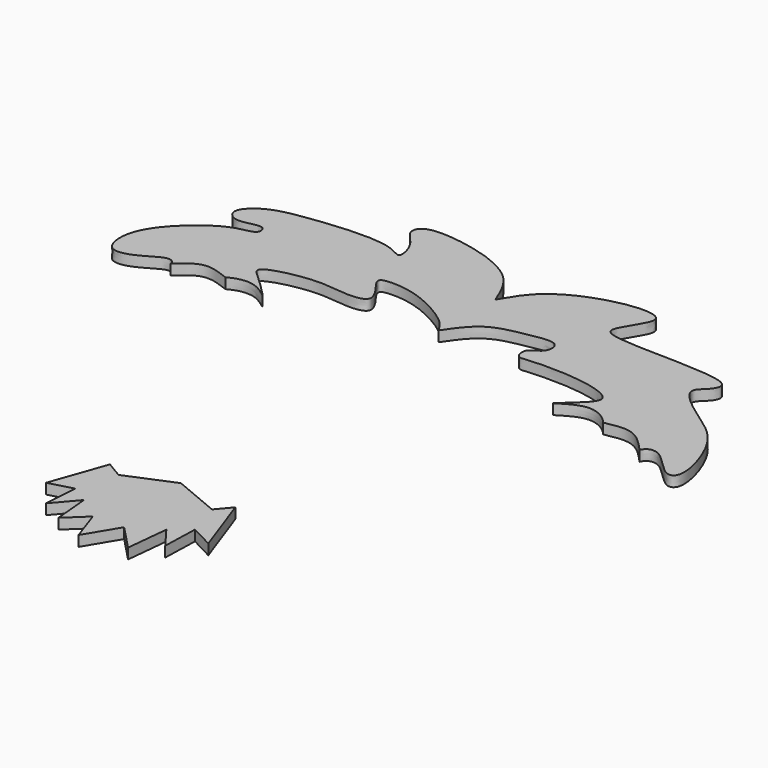
from build123d import *

# Parameters (mm, degrees)
F1_DEPTH = 2


# Not quite as in the source:
# - a feature of the source that left no trace in its solid (it failed there, or was rolled back) is left out


with BuildPart() as f1:
    # F0 (on Top) → F1 (new body)
    with BuildSketch(Plane.XY):
        with BuildLine():
            add(Edge.make_bspline(
                [(-78.1146883965, 32.7644832432), (-79.8439233254, 33.4284988046), (-83.278902367, 34.7475095986), (-85.9443386529, 32.3104507594), (-87.2679427266, 31.1002545059)],
                knots=[0, 0, 0, 0, 0.5034193536, 1, 1, 1, 1], degree=3))
            add(Edge.make_bspline(
                [(-42.5418205559, 39.2133668065), (-42.9881577653, 40.0131240327), (-44.1661912721, 42.1239514298), (-51.6115142204, 46.3650325189), (-57.0091765019, 47.0956703629), (-60.6148794703, 46.6201895743), (-57.7538294439, 43.4479557533), (-56.180778889, 40.1529498732), (-60.9940135931, 39.5538077388), (-66.3533249535, 40.8475728894), (-74.6350098706, 39.0417230977), (-76.3771578139, 37.4499603376), (-73.8439459206, 35.5138082715), (-68.5692401029, 30.1525469176), (-73.2253142698, 34.4011373863), (-76.557748644, 33.640558036), (-78.1146883965, 32.7644832432)],
                knots=[0, 0, 0, 0, 0.0469390695, 0.1238879383, 0.1885242015, 0.2276844615, 0.2763512093, 0.3210485779, 0.3702674052, 0.4367229163, 0.5131938234, 0.5454216494, 0.592150659, 0.651575906, 0.6989267584, 0.7597418512, 0.7597418512, 0.7597418512, 0.7597418512], degree=3))
            add(Edge.make_bspline(
                [(-4.6806400642, 31.308285892), (-5.9656620832, 32.847897371), (-9.6100700572, 35.0911827196), (-16.4039831582, 29.9517155128), (-11.2605175981, 34.3316004388), (-8.0465825383, 37.9134992605), (-16.4611236648, 40.442506288), (-25.7368132326, 40.2126806715), (-28.2032088922, 39.7228029764), (-28.753404739, 42.8519487562), (-25.6085695806, 43.4716036385), (-25.4385154838, 47.6426221355), (-31.7459644318, 46.3832888128), (-38.4448695025, 45.2151020848), (-41.1777001261, 41.2117040092), (-42.5418205559, 39.2133668065)],
                knots=[0.2054161527, 0.2054161527, 0.2054161527, 0.2054161527, 0.2744381238, 0.337088289, 0.3938683938, 0.4482000731, 0.5230968929, 0.6131068496, 0.6521978096, 0.6933793991, 0.7398666544, 0.78486673, 0.849818787, 0.9250355075, 1, 1, 1, 1], degree=3))
            add(Edge.make_bspline(
                [(-4.6806400642, 31.308285892), (-2.8738994377, 31.6778287409), (0.8586140408, 32.4412607711), (3.6542842794, 29.3610296947), (5.0966972485, 27.7717988938)],
                knots=[0, 0, 0, 0, 0.4840546824, 1, 1, 1, 1], degree=3))
            add(Edge.make_bspline(
                [(-42.1257652342, 52.3191578686), (-40.9383053307, 54.369264377), (-38.3302838513, 58.8719189874), (-28.8279433408, 63.1607793167), (-21.1409836142, 63.9358777675), (-18.3898677035, 61.946076837), (-22.6403519936, 56.6118059723), (-22.4195501027, 52.6678459901), (3.5197902884, 54.7494498371), (1.1236831442, 49.5189934563), (-2.3868660157, 47.461679138), (5.3601052781, 41.4084355763), (12.1001432584, 37.4360959792), (15.9557024653, 25.1871293377), (12.5633189349, 23.5096446907), (8.1180278163, 30.0136480103), (5.4226940702, 28.7641528644), (5.0966972485, 27.7717988938)],
                knots=[0, 0, 0, 0, 0.0673227732, 0.1478611935, 0.2162571792, 0.2520614536, 0.3134153549, 0.3507611814, 0.4692743729, 0.5087628221, 0.5507310653, 0.6197347319, 0.6957300099, 0.7786999902, 0.8127329943, 0.8785201714, 0.9195500013, 0.9195500013, 0.9195500013, 0.9195500013], degree=3))
            add(Edge.make_bspline(
                [(-87.2679427266, 31.1002545059), (-87.2485118161, 31.5557596075), (-88.5252620658, 33.0107379245), (-92.7033394549, 29.6531327281), (-98.0324174638, 28.49378586), (-99.0466215971, 35.0989526016), (-94.7272198386, 41.3863896024), (-87.764545452, 46.5886019068), (-82.9990861881, 46.6112042122), (-83.679558813, 49.797639546), (-88.405366619, 47.4283733088), (-91.4009523992, 50.330583999), (-87.6101072381, 54.195191634), (-80.6307891019, 55.6045445895), (-65.7166849924, 57.0841681174), (-61.5896949539, 53.3087577959), (-62.7642434778, 58.7416835725), (-66.1899903184, 61.1040883364), (-65.2347173459, 64.224795666), (-57.6081010337, 64.1981094362), (-45.4393527169, 60.6074817113), (-43.1537578364, 54.890490492), (-42.1257652342, 52.3191578686)],
                knots=[0.3781661826, 0.3781661826, 0.3781661826, 0.3781661826, 0.3948230743, 0.4256163056, 0.4543864352, 0.4847763275, 0.5229896191, 0.5637962148, 0.5903925864, 0.6072939236, 0.6360640538, 0.6590399339, 0.6864941146, 0.7247830495, 0.7783052081, 0.8024570428, 0.8286344533, 0.8566479295, 0.8759415404, 0.9119584894, 0.9604015469, 1, 1, 1, 1], degree=3))
        make_face()
    extrude(amount=F1_DEPTH)


with BuildPart() as f1b:
    # F0 (on Top) → F1, piece 2 (new body)
    with BuildSketch(Plane.XY):
        Polygon((-50.6549328566, -27.1477159113), (-53.7753589451, -25.2754576504), (-57.5198717415, -35.8849093318), (-52.9432445765, -34.6367396414), (-53.3593036234, -41.0856232047), (-49.614790827, -36.7170237005), (-48.9907041192, -43.5819625854), (-45.2461913228, -40.0454774499), (-43.1659072638, -46.0783056915), (-39.4213944674, -39.8374535143), (-34.8447673023, -44.622104615), (-34.0126529336, -36.5089960396), (-30.892226845, -40.6695641577), (-30.6841991842, -33.8046252728), (-26.3156015426, -36.0929407179), (-30.4761696607, -24.4433451444), (-32.7644832432, -27.1477159113), (-41.7097061872, -23.4032012522), align=None)
    extrude(amount=F1_DEPTH)


solid = Compound([f1.part, f1b.part])
